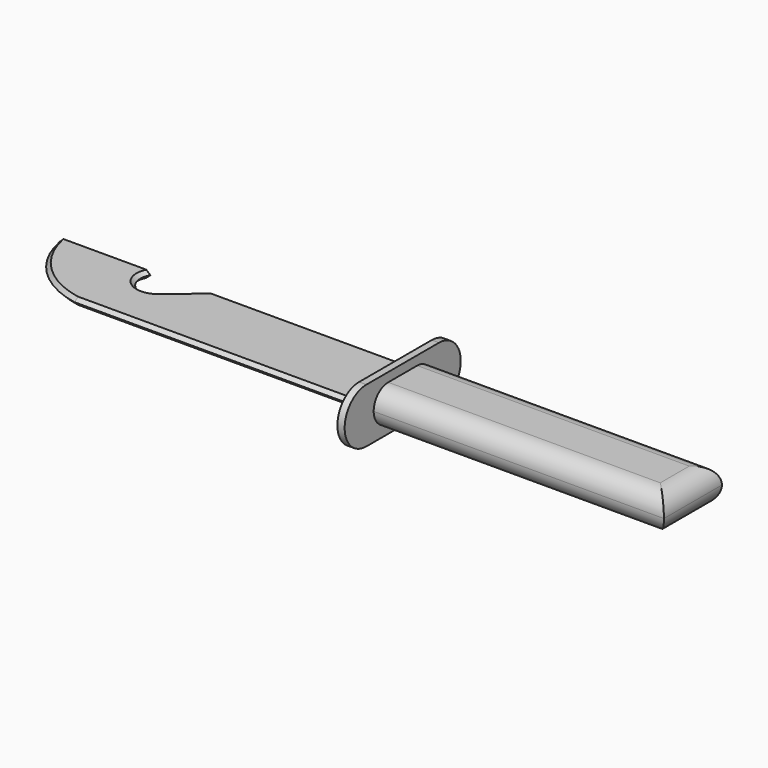
from build123d import *

# Parameters (mm, degrees)
F1_DEPTH   = 2.54
F2_C1_SIZE = 1.27
F2_C2_SIZE = 1.2699
F2_C3_SIZE = 1.27
F2_C4_SIZE = 1.2699
F3_SIZE    = 1.26999
F4_W       = 31.75
F4_H       = 19.05
F5_DEPTH   = 2.54
F6_W       = 25.4
F6_H       = 12.7
F7_DEPTH   = 101.6
F8_R       = 6.34999


# Not quite as in the source:
# - a fillet or chamfer is up to 0.001 mm smaller than in the source, because OpenCascade refuses the exact size


with BuildPart() as f1:
    # F0 (on Top) → F1 (new body)
    with BuildSketch(Plane.XY):
        with BuildLine():
            Line((31.75, 0), (0, 0))
            ThreePointArc((0, 0), (8.8381906554, -16.6839242395), (25.5862342852, -25.4))
            Line((25.5862342852, -25.4), (127.1862342852, -25.4))
            Line((127.1862342852, -25.4), (127.1862342852, 0))
            Line((127.1862342852, 0), (50.9862342852, 0))
            Line((50.9862342852, 0), (41.2574698576, -8.163402643))
            ThreePointArc((41.2574698576, -8.163402643), (33.0391135049, -8.1167569468), (31.75, 0))
        make_face()
    extrude(amount=F1_DEPTH)

    # F2: chamfer of 1.27 on 4 edges, made by hand

    # F2_c1
    f2_c1_edges = [f1.edges().sort_by_distance(p)[0] for p in [
        (76.3862342852, -25.4, 0),
    ]]
    chamfer(f2_c1_edges, length=F2_C1_SIZE)

    # F2_c2 (size 1.27 in the source; OpenCascade refuses exactly that, so slightly less here)
    f2_c2_edges = [f1.edges().sort_by_distance(p)[0] for p in [
        (76.3862342852, -25.4, 2.54),
    ]]
    chamfer(f2_c2_edges, length=F2_C2_SIZE)

    # F2_c3
    f2_c3_edges = [f1.edges().sort_by_distance(p)[0] for p in [
        (7.1332744951, -14.8524871452, 0),
    ]]
    chamfer(f2_c3_edges, length=F2_C3_SIZE)

    # F2_c4 (size 1.27 in the source; OpenCascade refuses exactly that, so slightly less here)
    f2_c4_edges = [f1.edges().sort_by_distance(p)[0] for p in [
        (7.133373479, -14.8526022537, 2.54),
    ]]
    chamfer(f2_c4_edges, length=F2_C4_SIZE)

    # F3 (size 1.27 in the source; OpenCascade refuses exactly that, so slightly less here)
    f3_edges = [f1.edges().sort_by_distance(p)[0] for p in [
        (33.039114, -8.116757, 0),
        (33.039114, -8.116757, 2.54),
        (46.121852, -4.081701, 0),
        (46.121852, -4.081701, 2.54),
    ]]
    chamfer(f3_edges, length=F3_SIZE)

    # F4 (on face) → F5 (join)
    with BuildSketch(Plane.YZ.offset(127.1862342852)):
        with Locations((-12.065, 1.27)):
            Rectangle(F4_W, F4_H)
        with BuildLine():
            ThreePointArc((3.81, -8.255), (13.335, 1.27), (3.81, 10.795))
            Line((3.81, 10.795), (3.81, -8.255))
        make_face()
        with BuildLine():
            Line((-27.94, -8.255), (-27.94, 10.795))
            ThreePointArc((-27.94, 10.795), (-37.465, 1.27), (-27.94, -8.255))
        make_face()
    extrude(amount=F5_DEPTH)

    # F6 (on face) → F7 (join)
    with BuildSketch(Plane.YZ.offset(129.7262342852)):
        with Locations((-12.065, 1.27)):
            Rectangle(F6_W, F6_H)
    extrude(amount=F7_DEPTH)

    # F8 (radius 6.35 in the source; OpenCascade refuses exactly that, so slightly less here)
    f8_edges = [f1.edges().sort_by_distance(p)[0] for p in [
        (180.526234, 0.635, 7.62),
        (180.526234, 0.635, -5.08),
        (180.526234, -24.765, -5.08),
        (180.526234, -24.765, 7.62),
        (231.326234, -12.065, 7.62),
        (231.326234, -12.065, -5.08),
    ]]
    fillet(f8_edges, radius=F8_R)


solid = f1.part
